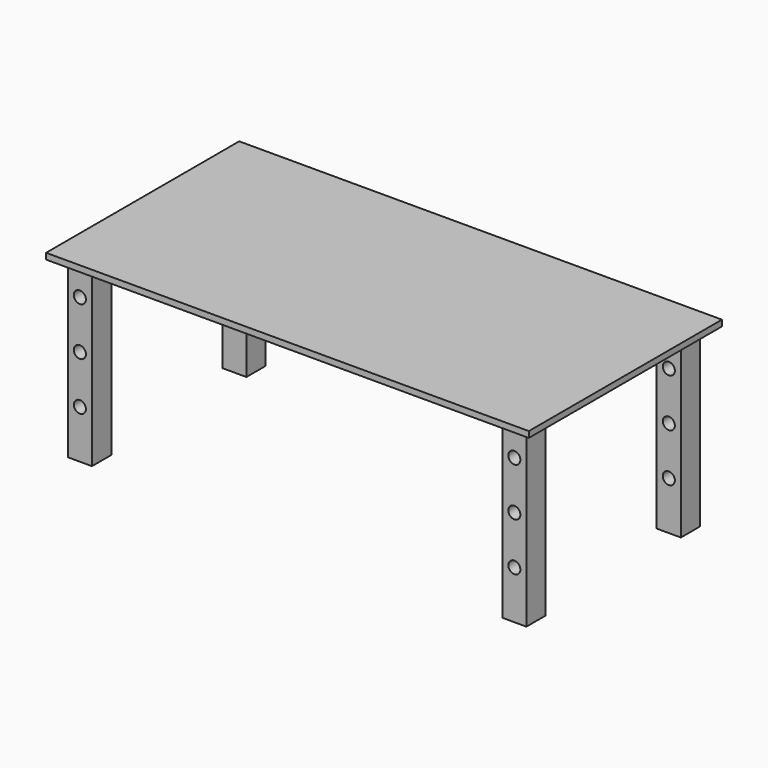
from build123d import *

# Parameters (mm, degrees)
F0_W      = 2000
F0_H      = 1000
F1_DEPTH  = 25
F2_W      = 100
F2_H      = 100
F3_DEPTH  = 725
F4_W      = 100
F4_H      = 100
F5_DEPTH  = 725
F6_W      = 100
F6_H      = 100
F7_DEPTH  = 725
F8_W      = 100
F8_H      = 100
F9_DEPTH  = 725
F10_R     = 25
F11_DEPTH = 1000.001
F12_R     = 25
F13_DEPTH = 1000.001


# Not quite as in the source:
# - a feature of the source that left no trace in its solid (it failed there, or was rolled back) is left out


with BuildPart() as f1:
    # F0 (on Top) → F1 (new body)
    with BuildSketch(Plane.XY):
        with Locations((1000, 500)):
            Rectangle(F0_W, F0_H)
    extrude(amount=F1_DEPTH)

    # F2 (on Top) → F3 (join)
    with BuildSketch(Plane.XY):
        with Locations((100, 100)):
            Rectangle(F2_W, F2_H)
    extrude(amount=-F3_DEPTH)

    # F4 (on Top) → F5 (join)
    with BuildSketch(Plane.XY):
        with Locations((1900, 100)):
            Rectangle(F4_W, F4_H)
    extrude(amount=-F5_DEPTH)

    # F6 (on Top) → F7 (join)
    with BuildSketch(Plane.XY):
        with Locations((100, 900)):
            Rectangle(F6_W, F6_H)
    extrude(amount=-F7_DEPTH)

    # F8 (on Top) → F9 (join)
    with BuildSketch(Plane.XY):
        with Locations((1900, 900)):
            Rectangle(F8_W, F8_H)
    extrude(amount=-F9_DEPTH)

    # F10 (on Front) → F11 (cut, through all)
    with BuildSketch(Plane.XZ):
        with Locations((100, -525)):
            Circle(F10_R)
        with Locations((100, -325)):
            Circle(F10_R)
        with Locations((100, -125)):
            Circle(F10_R)
    extrude(amount=-F11_DEPTH, mode=Mode.SUBTRACT)

    # F12 (on Front) → F13 (cut, through all)
    with BuildSketch(Plane.XZ):
        with Locations((1900, -525)):
            Circle(F12_R)
        with Locations((1900, -325)):
            Circle(F12_R)
        with Locations((1900, -125)):
            Circle(F12_R)
    extrude(amount=-F13_DEPTH, mode=Mode.SUBTRACT)


solid = f1.part
